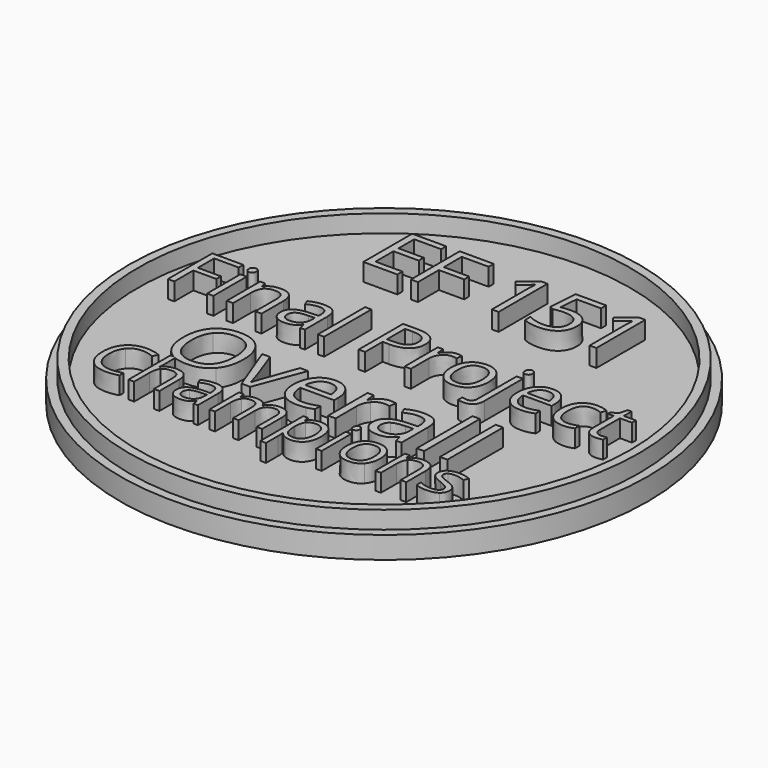
from build123d import *

# Parameters (mm, degrees)
F0_R           = 38.1
F1_DEPTH       = 3.175
F2_R           = 36.83
F2_R_2         = 35.56
F3_DEPTH       = 2.54
F4_TEXT_SIZE   = 12.3391885464
F4_TEXT_SIZE_2 = 11.2342395975
F4_W           = 1.0741905417
F4_H           = 10.0651032839
F4_W_2         = 0.8091592002
F4_H_2         = 5.3398270918
F5_DEPTH       = 2.54


# Not quite as in the source:
# - Text() gives the source's letters only with a copy of the font that has no kerning and outlines rounded to 1/6400 em; it was checked with that copy


with BuildPart() as f1:
    # F0 (on Top) → F1 (new body)
    with BuildSketch(Plane.XY):
        Circle(F0_R)
    extrude(amount=F1_DEPTH)

    # F2 (on face) → F3 (join)
    with BuildSketch(Plane.XY.offset(3.175)):
        Circle(F2_R)
        Circle(F2_R_2, mode=Mode.SUBTRACT)
    extrude(amount=F3_DEPTH)

    # F4 (on face) → F5 (join)
    with BuildSketch(Plane.XY.offset(3.175)):
        with Locations((-17.8262714532, 17.0286893845)):
            Text('EF 151', F4_TEXT_SIZE, font='Open Sans', text_align=(TextAlign.LEFT, TextAlign.BOTTOM))
        with Locations((-32.3159923422, 0)):
            Text('Final Project', F4_TEXT_SIZE_2, font='Open Sans', text_align=(TextAlign.LEFT, TextAlign.BOTTOM))
        with BuildLine():
            add(Edge.make_bspline(
                [(-12.2817855001, -10.0030932078), (-12.2817855001, -12.2735884376), (-13.4304863684, -13.5744145561)],
                knots=[0, 0, 0, 1, 1, 1], degree=2))
            add(Edge.make_bspline(
                [(-13.4263469058, -6.4328067252), (-12.2817855001, -7.7263887842), (-12.2817855001, -10.0030932078)],
                knots=[0, 0, 0, 1, 1, 1], degree=2))
            add(Edge.make_bspline(
                [(-16.6095936364, -5.1392246663), (-14.5709083115, -5.1392246663), (-13.4263469058, -6.4328067252)],
                knots=[0, 0, 0, 1, 1, 1], degree=2))
            add(Edge.make_bspline(
                [(-19.842513918, -6.410039681), (-18.7041617061, -5.1392246663), (-16.6095936364, -5.1392246663)],
                knots=[0, 0, 0, 1, 1, 1], degree=2))
            add(Edge.make_bspline(
                [(-20.9808661298, -9.9906748201), (-20.9808661298, -7.6808546957), (-19.842513918, -6.410039681)],
                knots=[0, 0, 0, 1, 1, 1], degree=2))
            add(Edge.make_bspline(
                [(-19.8456185149, -13.5971816003), (-20.9808661298, -12.3191225261), (-20.9808661298, -9.9906748201)],
                knots=[0, 0, 0, 1, 1, 1], degree=2))
            add(Edge.make_bspline(
                [(-18.9127607209, -14.3472838341), (-19.4400204931, -14.0538028919), (-19.8456185149, -13.5971816003)],
                knots=[0.6427228594, 0.6427228594, 0.6427228594, 1, 1, 1], degree=2))
            Line((-18.9127607209, -14.3472838341), (-18.5319283874, -14.3472838341))
            Line((-18.5319283874, -14.3472838341), (-18.5319283874, -14.5314262065))
            add(Edge.make_bspline(
                [(-16.6220120241, -14.8752406745), (-17.7051698515, -14.8752406745), (-18.5319283874, -14.5314262065)],
                knots=[0, 0, 0, 0.5186646031, 0.5186646031, 0.5186646031], degree=2))
            add(Edge.make_bspline(
                [(-13.4304863684, -13.5744145561), (-14.5791872367, -14.8752406745), (-16.6220120241, -14.8752406745)],
                knots=[0, 0, 0, 1, 1, 1], degree=2))
        make_face()
        with BuildLine():
            add(Edge.make_bspline(
                [(-19.8176771424, -10.0030932078), (-19.8176771424, -11.9238038489), (-18.9990984156, -12.9172748701)],
                knots=[0, 0, 0, 1, 1, 1], degree=2))
            add(Edge.make_bspline(
                [(-18.9990984156, -7.1158180523), (-19.8176771424, -8.1092890736), (-19.8176771424, -10.0030932078)],
                knots=[0, 0, 0, 1, 1, 1], degree=2))
            add(Edge.make_bspline(
                [(-16.6095936364, -6.1223470311), (-18.1805196887, -6.1223470311), (-18.9990984156, -7.1158180523)],
                knots=[0, 0, 0, 1, 1, 1], degree=2))
            add(Edge.make_bspline(
                [(-14.2459604983, -7.1085739928), (-15.0448767779, -6.1223470311), (-16.6095936364, -6.1223470311)],
                knots=[0, 0, 0, 1, 1, 1], degree=2))
            add(Edge.make_bspline(
                [(-13.4470442187, -10.0030932078), (-13.4470442187, -8.0948009545), (-14.2459604983, -7.1085739928)],
                knots=[0, 0, 0, 1, 1, 1], degree=2))
            add(Edge.make_bspline(
                [(-14.2490650953, -12.9214143327), (-13.4470442187, -11.9320827741), (-13.4470442187, -10.0030932078)],
                knots=[0, 0, 0, 1, 1, 1], degree=2))
            add(Edge.make_bspline(
                [(-16.6220120241, -13.9107458914), (-15.0510859718, -13.9107458914), (-14.2490650953, -12.9214143327)],
                knots=[0, 0, 0, 1, 1, 1], degree=2))
            add(Edge.make_bspline(
                [(-18.9990984156, -12.9172748701), (-18.1805196887, -13.9107458914), (-16.6220120241, -13.9107458914)],
                knots=[0, 0, 0, 1, 1, 1], degree=2))
        make_face(mode=Mode.SUBTRACT)
        with BuildLine():
            Line((-18.5319283874, -16.6422401784), (-18.5319283874, -14.5314262065))
            add(Edge.make_bspline(
                [(-18.5319283874, -14.5314262065), (-18.7296789602, -14.449189973), (-18.9127607209, -14.3472838341)],
                knots=[0.5186646031, 0.5186646031, 0.5186646031, 0.6427228594, 0.6427228594, 0.6427228594], degree=2))
            Line((-18.9127607209, -14.3472838341), (-19.3410875876, -14.3472838341))
            Line((-19.3410875876, -14.3472838341), (-19.3410875876, -21.9290587677))
            Line((-19.3410875876, -21.9290587677), (-18.5319283874, -21.9290587677))
            Line((-18.5319283874, -21.9290587677), (-18.5319283874, -19.1367579439))
            add(Edge.make_bspline(
                [(-18.144498597, -17.6369291374), (-18.5319283874, -18.0952967768), (-18.5319283874, -19.1367579439)],
                knots=[0, 0, 0, 1, 1, 1], degree=2))
            add(Edge.make_bspline(
                [(-16.9151690607, -17.1785614979), (-17.7570688065, -17.1785614979), (-18.144498597, -17.6369291374)],
                knots=[0, 0, 0, 1, 1, 1], degree=2))
            add(Edge.make_bspline(
                [(-15.9836225826, -17.5005101971), (-16.2806261041, -17.1785614979), (-16.9151690607, -17.1785614979)],
                knots=[0, 0, 0, 1, 1, 1], degree=2))
            add(Edge.make_bspline(
                [(-15.6866190611, -18.4741516624), (-15.6866190611, -17.8224588962), (-15.9836225826, -17.5005101971)],
                knots=[0, 0, 0, 1, 1, 1], degree=2))
            Line((-15.6866190611, -18.4741516624), (-15.6866190611, -21.9290587677))
            Line((-15.6866190611, -21.9290587677), (-14.877459861, -21.9290587677))
            Line((-14.877459861, -21.9290587677), (-14.877459861, -18.4460883376))
            add(Edge.make_bspline(
                [(-15.3677885092, -16.9673070247), (-14.877459861, -17.4326904953), (-14.877459861, -18.4460883376)],
                knots=[0, 0, 0, 1, 1, 1], degree=2))
            add(Edge.make_bspline(
                [(-16.8372153805, -16.501923554), (-15.8581171575, -16.501923554), (-15.3677885092, -16.9673070247)],
                knots=[0, 0, 0, 1, 1, 1], degree=2))
            add(Edge.make_bspline(
                [(-17.8428178547, -16.7233120057), (-17.4016000249, -16.501923554), (-16.8372153805, -16.501923554)],
                knots=[0, 0, 0, 1, 1, 1], degree=2))
            add(Edge.make_bspline(
                [(-18.5225739458, -17.3297916375), (-18.2840356845, -16.9447004574), (-17.8428178547, -16.7233120057)],
                knots=[0, 0, 0, 1, 1, 1], degree=2))
            Line((-18.5225739458, -17.3297916375), (-18.5709052275, -17.3297916375))
            add(Edge.make_bspline(
                [(-18.5319283874, -16.6422401784), (-18.5319283874, -17.0569537569), (-18.5709052275, -17.3297916375)],
                knots=[0, 0, 0, 1, 1, 1], degree=2))
        make_face()
        with BuildLine():
            add(Edge.make_bspline(
                [(-18.5319283874, -14.5314262065), (-18.7296789602, -14.449189973), (-18.9127607209, -14.3472838341)],
                knots=[0.5186646031, 0.5186646031, 0.5186646031, 0.6427228594, 0.6427228594, 0.6427228594], degree=2))
            Line((-18.5319283874, -14.5314262065), (-18.5319283874, -14.3472838341))
            Line((-18.5319283874, -14.3472838341), (-18.9127607209, -14.3472838341))
        make_face()
        with BuildLine():
            Line((-11.4745902953, -7.6560179201), (-8.7839396128, -14.744847603))
            Line((-8.7839396128, -14.744847603), (-7.5296824485, -14.744847603))
            Line((-7.5296824485, -14.744847603), (-4.839031766, -7.6560179201))
            Line((-4.839031766, -7.6560179201), (-5.9898023656, -7.6560179201))
            add(Edge.make_bspline(
                [(-7.6869820268, -12.3553428237), (-7.3082212, -11.2780476851), (-5.9898023656, -7.6560179201)],
                knots=[0, 0, 0, 1, 1, 1], degree=2))
            add(Edge.make_bspline(
                [(-8.1361137177, -13.774143626), (-8.0657428537, -13.4326379624), (-7.6869820268, -12.3553428237)],
                knots=[0, 0, 0, 1, 1, 1], degree=2))
            Line((-8.1361137177, -13.774143626), (-8.1878570001, -13.774143626))
            add(Edge.make_bspline(
                [(-8.7963580006, -11.8596421788), (-8.278925177, -13.3353605916), (-8.1878570001, -13.774143626)],
                knots=[0, 0, 0, 1, 1, 1], degree=2))
            Line((-8.7963580006, -11.8596421788), (-10.3238196957, -7.6560179201))
            Line((-10.3238196957, -7.6560179201), (-11.4745902953, -7.6560179201))
        make_face()
        with BuildLine():
            add(Edge.make_bspline(
                [(-0.7057783713, -14.8752406745), (-2.2767044237, -14.8752406745), (-3.1863513275, -13.9169550853)],
                knots=[0, 0, 0, 1, 1, 1], degree=2))
            add(Edge.make_bspline(
                [(0.5195025549, -14.7676146472), (0.0124183878, -14.8752406745), (-0.7057783713, -14.8752406745)],
                knots=[0, 0, 0, 1, 1, 1], degree=2))
            add(Edge.make_bspline(
                [(1.5957628279, -14.4157603272), (1.0265867219, -14.6599886199), (0.5195025549, -14.7676146472)],
                knots=[0, 0, 0, 1, 1, 1], degree=2))
            Line((1.5957628279, -14.4157603272), (1.5957628279, -13.4574747379))
            add(Edge.make_bspline(
                [(-0.6664534767, -13.9355826669), (0.478107929, -13.9355826669), (1.5957628279, -13.4574747379)],
                knots=[0, 0, 0, 1, 1, 1], degree=2))
            add(Edge.make_bspline(
                [(-2.3512147503, -13.2887916374), (-1.7530624062, -13.9355826669), (-0.6664534767, -13.9355826669)],
                knots=[0, 0, 0, 1, 1, 1], degree=2))
            add(Edge.make_bspline(
                [(-2.982482795, -11.3939526376), (-2.9493670943, -12.642000608), (-2.3512147503, -13.2887916374)],
                knots=[0, 0, 0, 1, 1, 1], degree=2))
            Line((-2.982482795, -11.3939526376), (1.9000133281, -11.3939526376))
            Line((1.9000133281, -11.3939526376), (1.9000133281, -10.715080773))
            add(Edge.make_bspline(
                [(1.1238640928, -8.4021560517), (1.9000133281, -9.2786872548), (1.9000133281, -10.715080773)],
                knots=[0, 0, 0, 1, 1, 1], degree=2))
            add(Edge.make_bspline(
                [(-0.9831223648, -7.5256248486), (0.3477148574, -7.5256248486), (1.1238640928, -8.4021560517)],
                knots=[0, 0, 0, 1, 1, 1], degree=2))
            add(Edge.make_bspline(
                [(-3.2515478633, -8.5346188546), (-2.4070974952, -7.5256248486), (-0.9831223648, -7.5256248486)],
                knots=[0, 0, 0, 1, 1, 1], degree=2))
            add(Edge.make_bspline(
                [(-4.0959982313, -11.2594201034), (-4.0959982313, -9.5436128605), (-3.2515478633, -8.5346188546)],
                knots=[0, 0, 0, 1, 1, 1], degree=2))
            add(Edge.make_bspline(
                [(-3.1863513275, -13.9169550853), (-4.0959982313, -12.958669496), (-4.0959982313, -11.2594201034)],
                knots=[0, 0, 0, 1, 1, 1], degree=2))
        make_face()
        with BuildLine():
            add(Edge.make_bspline(
                [(-0.9976104838, -8.4259579616), (-1.8503397771, -8.4259579616), (-2.3584588098, -8.9816808141)],
                knots=[0, 0, 0, 1, 1, 1], degree=2))
            add(Edge.make_bspline(
                [(0.2970064407, -8.9661578294), (-0.1552298471, -8.4259579616), (-0.9976104838, -8.4259579616)],
                knots=[0, 0, 0, 1, 1, 1], degree=2))
            add(Edge.make_bspline(
                [(0.7492427285, -10.5205260314), (0.7492427285, -9.5063576972), (0.2970064407, -8.9661578294)],
                knots=[0, 0, 0, 1, 1, 1], degree=2))
            Line((0.7492427285, -10.5205260314), (-2.9576460195, -10.5205260314))
            add(Edge.make_bspline(
                [(-2.3584588098, -8.9816808141), (-2.8665778425, -9.5374036666), (-2.9576460195, -10.5205260314)],
                knots=[0, 0, 0, 1, 1, 1], degree=2))
        make_face(mode=Mode.SUBTRACT)
        with BuildLine():
            add(Edge.make_bspline(
                [(6.9667155364, -7.5256248486), (7.4386142715, -7.5256248486), (7.8132356358, -7.6042746378)],
                knots=[0, 0, 0, 1, 1, 1], degree=2))
            add(Edge.make_bspline(
                [(5.7435043415, -7.9012810785), (6.3002620597, -7.5256248486), (6.9667155364, -7.5256248486)],
                knots=[0, 0, 0, 1, 1, 1], degree=2))
            add(Edge.make_bspline(
                [(4.7934976775, -8.9682275607), (5.1867466234, -8.2769373084), (5.7435043415, -7.9012810785)],
                knots=[0, 0, 0, 1, 1, 1], degree=2))
            Line((4.7934976775, -8.9682275607), (4.7417543951, -8.9682275607))
            Line((4.7417543951, -8.9682275607), (4.6175705175, -7.6560179201))
            Line((4.6175705175, -7.6560179201), (3.7317255235, -7.6560179201))
            Line((3.7317255235, -7.6560179201), (3.7317255235, -14.744847603))
            Line((3.7317255235, -14.744847603), (4.8059160652, -14.744847603))
            Line((4.8059160652, -14.744847603), (4.8059160652, -10.9406814841))
            add(Edge.make_bspline(
                [(5.4164867971, -9.2010723313), (4.8059160652, -9.8996066431), (4.8059160652, -10.9406814841)],
                knots=[0, 0, 0, 1, 1, 1], degree=2))
            add(Edge.make_bspline(
                [(6.8880657473, -8.5025380195), (6.0270575289, -8.5025380195), (5.4164867971, -9.2010723313)],
                knots=[0, 0, 0, 1, 1, 1], degree=2))
            add(Edge.make_bspline(
                [(7.6642149826, -8.5998153903), (7.2254319482, -8.5025380195), (6.8880657473, -8.5025380195)],
                knots=[0, 0, 0, 1, 1, 1], degree=2))
            Line((7.6642149826, -8.5998153903), (7.8132356358, -7.6042746378))
        make_face()
        with BuildLine():
            Line((13.2856051778, -13.7348187314), (13.4987875011, -14.744847603))
            Line((13.4987875011, -14.744847603), (14.2956340494, -14.744847603))
            Line((14.2956340494, -14.744847603), (14.2956340494, -9.905815837))
            add(Edge.make_bspline(
                [(13.6840284519, -8.1020450141), (14.2956340494, -8.6639770604), (14.2956340494, -9.905815837)],
                knots=[0, 0, 0, 1, 1, 1], degree=2))
            add(Edge.make_bspline(
                [(11.8057473024, -7.5401129677), (13.0724228545, -7.5401129677), (13.6840284519, -8.1020450141)],
                knots=[0, 0, 0, 1, 1, 1], degree=2))
            add(Edge.make_bspline(
                [(10.5525250037, -7.7015520086), (11.1765489889, -7.5401129677), (11.8057473024, -7.5401129677)],
                knots=[0, 0, 0, 1, 1, 1], degree=2))
            add(Edge.make_bspline(
                [(9.4048590011, -8.1465442369), (9.9285010185, -7.8629910496), (10.5525250037, -7.7015520086)],
                knots=[0, 0, 0, 1, 1, 1], degree=2))
            Line((9.4048590011, -8.1465442369), (9.7360160082, -8.9682275607))
            add(Edge.make_bspline(
                [(11.739515901, -8.4259579616), (10.853670907, -8.4259579616), (9.7360160082, -8.9682275607)],
                knots=[0, 0, 0, 1, 1, 1], degree=2))
            add(Edge.make_bspline(
                [(12.8882167693, -8.8233463701), (12.5301532554, -8.4259579616), (11.739515901, -8.4259579616)],
                knots=[0, 0, 0, 1, 1, 1], degree=2))
            add(Edge.make_bspline(
                [(13.2462802832, -10.0548364902), (13.2462802832, -9.2207347786), (12.8882167693, -8.8233463701)],
                knots=[0, 0, 0, 1, 1, 1], degree=2))
            Line((13.2462802832, -10.0548364902), (13.2462802832, -10.4956892559))
            Line((13.2462802832, -10.4956892559), (12.0437664012, -10.5350141505))
            add(Edge.make_bspline(
                [(8.6100821841, -12.7848120673), (8.6100821841, -10.6385007152), (12.0437664012, -10.5350141505)],
                knots=[0, 0, 0, 1, 1, 1], degree=2))
            add(Edge.make_bspline(
                [(9.2082345281, -14.3309013441), (8.6100821841, -13.7865620137), (8.6100821841, -12.7848120673)],
                knots=[0, 0, 0, 1, 1, 1], degree=2))
            add(Edge.make_bspline(
                [(10.8598801009, -14.8752406745), (9.8063868722, -14.8752406745), (9.2082345281, -14.3309013441)],
                knots=[0, 0, 0, 1, 1, 1], degree=2))
            add(Edge.make_bspline(
                [(12.1772640697, -14.6382564413), (11.6505174553, -14.8752406745), (10.8598801009, -14.8752406745)],
                knots=[0, 0, 0, 1, 1, 1], degree=2))
            add(Edge.make_bspline(
                [(13.2338618954, -13.7348187314), (12.7040106841, -14.4012722081), (12.1772640697, -14.6382564413)],
                knots=[0, 0, 0, 1, 1, 1], degree=2))
            Line((13.2338618954, -13.7348187314), (13.2856051778, -13.7348187314))
        make_face()
        with BuildLine():
            add(Edge.make_bspline(
                [(11.0730624242, -13.9873259493), (12.0768821019, -13.9873259493), (12.6491628048, -13.4378122906)],
                knots=[0, 0, 0, 1, 1, 1], degree=2))
            add(Edge.make_bspline(
                [(10.0878703282, -13.6841103147), (10.4397246482, -13.9873259493), (11.0730624242, -13.9873259493)],
                knots=[0, 0, 0, 1, 1, 1], degree=2))
            add(Edge.make_bspline(
                [(9.7360160082, -12.7972304551), (9.7360160082, -13.38089468), (10.0878703282, -13.6841103147)],
                knots=[0, 0, 0, 1, 1, 1], degree=2))
            add(Edge.make_bspline(
                [(10.3010526515, -11.7013077348), (9.7360160082, -12.0541969204), (9.7360160082, -12.7972304551)],
                knots=[0, 0, 0, 1, 1, 1], degree=2))
            add(Edge.make_bspline(
                [(12.147252966, -11.3028844606), (10.8660892948, -11.3484185491), (10.3010526515, -11.7013077348)],
                knots=[0, 0, 0, 1, 1, 1], degree=2))
            Line((12.147252966, -11.3028844606), (13.2214435077, -11.2594201034))
            Line((13.2214435077, -11.2594201034), (13.2214435077, -11.8989670734))
            add(Edge.make_bspline(
                [(12.6491628048, -13.4378122906), (13.2214435077, -12.888298632), (13.2214435077, -11.8989670734)],
                knots=[0, 0, 0, 1, 1, 1], degree=2))
        make_face(mode=Mode.SUBTRACT)
        with Locations((17.0432023425, -9.712295961)):
            Rectangle(F4_W, F4_H)
        with Locations((20.3940973079, -9.712295961)):
            Rectangle(F4_W, F4_H)
        with BuildLine():
            add(Edge.make_bspline(
                [(-22.465471089, -15.4448716509), (-23.6394535124, -15.4448716509), (-24.3192096035, -16.226747063)],
                knots=[0, 0, 0, 1, 1, 1], degree=2))
            add(Edge.make_bspline(
                [(-20.8471526886, -15.8237265365), (-21.6563118888, -15.4448716509), (-22.465471089, -15.4448716509)],
                knots=[0, 0, 0, 1, 1, 1], degree=2))
            Line((-20.8471526886, -15.8237265365), (-20.4963611278, -15.1127889734))
            add(Edge.make_bspline(
                [(-22.4545575737, -14.7043116893), (-21.3351427265, -14.7043116893), (-20.4963611278, -15.1127889734)],
                knots=[0, 0, 0, 1, 1, 1], degree=2))
            add(Edge.make_bspline(
                [(-24.2841304474, -15.1525453503), (-23.5069322561, -14.7043116893), (-22.4545575737, -14.7043116893)],
                knots=[0, 0, 0, 1, 1, 1], degree=2))
            add(Edge.make_bspline(
                [(-25.47292407, -16.4286470947), (-25.0613286387, -15.6007790113), (-24.2841304474, -15.1525453503)],
                knots=[0, 0, 0, 1, 1, 1], degree=2))
            add(Edge.make_bspline(
                [(-25.8845195013, -18.3572211422), (-25.8845195013, -17.2565151781), (-25.47292407, -16.4286470947)],
                knots=[0, 0, 0, 1, 1, 1], degree=2))
            add(Edge.make_bspline(
                [(-25.0293676298, -21.0715682858), (-25.8845195013, -20.1158561669), (-25.8845195013, -18.3572211422)],
                knots=[0, 0, 0, 1, 1, 1], degree=2))
            add(Edge.make_bspline(
                [(-22.6011104925, -22.0272804047), (-24.1742157583, -22.0272804047), (-25.0293676298, -21.0715682858)],
                knots=[0, 0, 0, 1, 1, 1], degree=2))
            add(Edge.make_bspline(
                [(-20.7738762292, -21.7482062297), (-21.5144361909, -22.0272804047), (-22.6011104925, -22.0272804047)],
                knots=[0, 0, 0, 1, 1, 1], degree=2))
            Line((-20.7738762292, -21.7482062297), (-20.7738762292, -21.0232370041))
            add(Edge.make_bspline(
                [(-22.4748255306, -21.2913976639), (-21.7295883481, -21.2913976639), (-20.7738762292, -21.0232370041)],
                knots=[0, 0, 0, 1, 1, 1], degree=2))
            add(Edge.make_bspline(
                [(-24.3433752443, -20.528231135), (-23.6877847941, -21.2913976639), (-22.4748255306, -21.2913976639)],
                knots=[0, 0, 0, 1, 1, 1], degree=2))
            add(Edge.make_bspline(
                [(-24.9989656946, -18.3681346574), (-24.9989656946, -19.7650646061), (-24.3433752443, -20.528231135)],
                knots=[0, 0, 0, 1, 1, 1], degree=2))
            add(Edge.make_bspline(
                [(-24.3192096035, -16.226747063), (-24.9989656946, -17.0086224752), (-24.9989656946, -18.3681346574)],
                knots=[0, 0, 0, 1, 1, 1], degree=2))
        make_face()
        with BuildLine():
            Line((-10.0942220456, -21.1682308492), (-9.9336374644, -21.9290587677))
            Line((-9.9336374644, -21.9290587677), (-9.3333941271, -21.9290587677))
            Line((-9.3333941271, -21.9290587677), (-9.3333941271, -18.2839446828))
            add(Edge.make_bspline(
                [(-9.7941003769, -16.9252120374), (-9.3333941271, -17.3485005207), (-9.3333941271, -18.2839446828)],
                knots=[0, 0, 0, 1, 1, 1], degree=2))
            add(Edge.make_bspline(
                [(-11.208959672, -16.501923554), (-10.2548066267, -16.501923554), (-9.7941003769, -16.9252120374)],
                knots=[0, 0, 0, 1, 1, 1], degree=2))
            add(Edge.make_bspline(
                [(-12.1529787389, -16.6235312951), (-11.6829180475, -16.501923554), (-11.208959672, -16.501923554)],
                knots=[0, 0, 0, 1, 1, 1], degree=2))
            add(Edge.make_bspline(
                [(-13.017485052, -16.9587321199), (-12.6230394304, -16.7451390362), (-12.1529787389, -16.6235312951)],
                knots=[0, 0, 0, 1, 1, 1], degree=2))
            Line((-13.017485052, -16.9587321199), (-12.7680332755, -17.5776843404))
            add(Edge.make_bspline(
                [(-11.2588500273, -17.1692070563), (-11.9261335296, -17.1692070563), (-12.7680332755, -17.5776843404)],
                knots=[0, 0, 0, 1, 1, 1], degree=2))
            add(Edge.make_bspline(
                [(-10.3935641774, -17.4685491882), (-10.6632839108, -17.1692070563), (-11.2588500273, -17.1692070563)],
                knots=[0, 0, 0, 1, 1, 1], degree=2))
            add(Edge.make_bspline(
                [(-10.123844444, -18.3961979822), (-10.123844444, -17.7678913201), (-10.3935641774, -17.4685491882)],
                knots=[0, 0, 0, 1, 1, 1], degree=2))
            Line((-10.123844444, -18.3961979822), (-10.123844444, -18.7282806598))
            Line((-10.123844444, -18.7282806598), (-11.0296662076, -18.7579030582))
            add(Edge.make_bspline(
                [(-13.6161693158, -20.4526160652), (-13.6161693158, -18.8358567384), (-11.0296662076, -18.7579030582)],
                knots=[0, 0, 0, 1, 1, 1], degree=2))
            add(Edge.make_bspline(
                [(-13.1655970444, -21.617244047), (-13.6161693158, -21.2072076893), (-13.6161693158, -20.4526160652)],
                knots=[0, 0, 0, 1, 1, 1], degree=2))
            add(Edge.make_bspline(
                [(-11.9214563088, -22.0272804047), (-12.715024773, -22.0272804047), (-13.1655970444, -21.617244047)],
                knots=[0, 0, 0, 1, 1, 1], degree=2))
            add(Edge.make_bspline(
                [(-10.9291059602, -21.8487664771), (-11.3258901923, -22.0272804047), (-11.9214563088, -22.0272804047)],
                knots=[0, 0, 0, 1, 1, 1], degree=2))
            add(Edge.make_bspline(
                [(-10.1331988856, -21.1682308492), (-10.5323217281, -21.6702525495), (-10.9291059602, -21.8487664771)],
                knots=[0, 0, 0, 1, 1, 1], degree=2))
            Line((-10.1331988856, -21.1682308492), (-10.0942220456, -21.1682308492))
        make_face()
        with BuildLine():
            add(Edge.make_bspline(
                [(-11.7608717277, -21.3584378288), (-11.00472103, -21.3584378288), (-10.5736371786, -20.9445037871)],
                knots=[0, 0, 0, 1, 1, 1], degree=2))
            add(Edge.make_bspline(
                [(-12.5029907629, -21.1300335459), (-12.2379482503, -21.3584378288), (-11.7608717277, -21.3584378288)],
                knots=[0, 0, 0, 1, 1, 1], degree=2))
            add(Edge.make_bspline(
                [(-12.7680332755, -20.4619705068), (-12.7680332755, -20.901629263), (-12.5029907629, -21.1300335459)],
                knots=[0, 0, 0, 1, 1, 1], degree=2))
            add(Edge.make_bspline(
                [(-12.3424061817, -19.6364410338), (-12.7680332755, -19.9022630832), (-12.7680332755, -20.4619705068)],
                knots=[0, 0, 0, 1, 1, 1], degree=2))
            add(Edge.make_bspline(
                [(-10.9517125275, -19.3363193651), (-11.916779088, -19.3706189844), (-12.3424061817, -19.6364410338)],
                knots=[0, 0, 0, 1, 1, 1], degree=2))
            Line((-10.9517125275, -19.3363193651), (-10.1425533273, -19.3035788195))
            Line((-10.1425533273, -19.3035788195), (-10.1425533273, -19.7853325629))
            add(Edge.make_bspline(
                [(-10.5736371786, -20.9445037871), (-10.1425533273, -20.5305697454), (-10.1425533273, -19.7853325629)],
                knots=[0, 0, 0, 1, 1, 1], degree=2))
        make_face(mode=Mode.SUBTRACT)
        with BuildLine():
            Line((-0.8613881659, -18.4554427792), (-0.8613881659, -21.9290587677))
            Line((-0.8613881659, -21.9290587677), (-0.0537880393, -21.9290587677))
            Line((-0.0537880393, -21.9290587677), (-0.0537880393, -18.4460883376))
            add(Edge.make_bspline(
                [(-0.5043603107, -16.9563935095), (-0.0537880393, -17.4217769801), (-0.0537880393, -18.4460883376)],
                knots=[0, 0, 0, 1, 1, 1], degree=2))
            add(Edge.make_bspline(
                [(-1.8607543457, -16.4910100388), (-0.9549325821, -16.4910100388), (-0.5043603107, -16.9563935095)],
                knots=[0, 0, 0, 1, 1, 1], degree=2))
            add(Edge.make_bspline(
                [(-2.893640608, -16.7350050578), (-2.4407297262, -16.4910100388), (-1.8607543457, -16.4910100388)],
                knots=[0, 0, 0, 1, 1, 1], degree=2))
            add(Edge.make_bspline(
                [(-3.5850897511, -17.398390876), (-3.3465514898, -16.9790000767), (-2.893640608, -16.7350050578)],
                knots=[0, 0, 0, 1, 1, 1], degree=2))
            Line((-3.5850897511, -17.398390876), (-3.6240665912, -17.398390876))
            add(Edge.make_bspline(
                [(-5.2610938749, -16.4910100388), (-4.0091577713, -16.4910100388), (-3.6240665912, -17.398390876)],
                knots=[0, 0, 0, 1, 1, 1], degree=2))
            add(Edge.make_bspline(
                [(-6.1941994265, -16.7108394169), (-5.7771472376, -16.4910100388), (-5.2610938749, -16.4910100388)],
                knots=[0, 0, 0, 1, 1, 1], degree=2))
            add(Edge.make_bspline(
                [(-6.8404354352, -17.3204371959), (-6.6112516154, -16.930668795), (-6.1941994265, -16.7108394169)],
                knots=[0, 0, 0, 1, 1, 1], degree=2))
            Line((-6.8404354352, -17.3204371959), (-6.8794122752, -17.3204371959))
            Line((-6.8794122752, -17.3204371959), (-7.0103744579, -16.5892316758))
            Line((-7.0103744579, -16.5892316758), (-7.6683035186, -16.5892316758))
            Line((-7.6683035186, -16.5892316758), (-7.6683035186, -21.9290587677))
            Line((-7.6683035186, -21.9290587677), (-6.8591443184, -21.9290587677))
            Line((-6.8591443184, -21.9290587677), (-6.8591443184, -19.1274035023))
            add(Edge.make_bspline(
                [(-6.5060141472, -17.6338109902), (-6.8591443184, -18.0890604824), (-6.8591443184, -19.1274035023)],
                knots=[0, 0, 0, 1, 1, 1], degree=2))
            add(Edge.make_bspline(
                [(-5.3936151311, -17.1785614979), (-6.152883976, -17.1785614979), (-6.5060141472, -17.6338109902)],
                knots=[0, 0, 0, 1, 1, 1], degree=2))
            add(Edge.make_bspline(
                [(-4.5408018701, -17.4973920499), (-4.8136397507, -17.1785614979), (-5.3936151311, -17.1785614979)],
                knots=[0, 0, 0, 1, 1, 1], degree=2))
            add(Edge.make_bspline(
                [(-4.2679639895, -18.4554427792), (-4.2679639895, -17.8162226018), (-4.5408018701, -17.4973920499)],
                knots=[0, 0, 0, 1, 1, 1], degree=2))
            Line((-4.2679639895, -18.4554427792), (-4.2679639895, -21.9290587677))
            Line((-4.2679639895, -21.9290587677), (-3.4588047893, -21.9290587677))
            Line((-3.4588047893, -21.9290587677), (-3.4588047893, -18.9465509643))
            add(Edge.make_bspline(
                [(-3.0978792501, -17.6119839597), (-3.4588047893, -18.0454064215), (-3.4588047893, -18.9465509643)],
                knots=[0, 0, 0, 1, 1, 1], degree=2))
            add(Edge.make_bspline(
                [(-1.9823620868, -17.1785614979), (-2.7369537109, -17.1785614979), (-3.0978792501, -17.6119839597)],
                knots=[0, 0, 0, 1, 1, 1], degree=2))
            add(Edge.make_bspline(
                [(-1.1342260465, -17.4973920499), (-1.4070639271, -17.1785614979), (-1.9823620868, -17.1785614979)],
                knots=[0, 0, 0, 1, 1, 1], degree=2))
            add(Edge.make_bspline(
                [(-0.8613881659, -18.4554427792), (-0.8613881659, -17.8162226018), (-1.1342260465, -17.4973920499)],
                knots=[0, 0, 0, 1, 1, 1], degree=2))
        make_face()
        with BuildLine():
            add(Edge.make_bspline(
                [(4.0980249667, -22.0272804047), (3.5757353095, -22.0272804047), (3.1446514582, -21.8347348147)],
                knots=[0, 0, 0, 1, 1, 1], degree=2))
            add(Edge.make_bspline(
                [(5.7280364191, -21.2984134951), (5.1410452074, -22.0272804047), (4.0980249667, -22.0272804047)],
                knots=[0, 0, 0, 1, 1, 1], degree=2))
            add(Edge.make_bspline(
                [(6.3150276308, -19.2536884641), (6.3150276308, -20.5695465855), (5.7280364191, -21.2984134951)],
                knots=[0, 0, 0, 1, 1, 1], degree=2))
            add(Edge.make_bspline(
                [(5.7373908607, -17.217538338), (6.3150276308, -17.9440666372), (6.3150276308, -19.2536884641)],
                knots=[0, 0, 0, 1, 1, 1], degree=2))
            add(Edge.make_bspline(
                [(4.0980249667, -16.4910100388), (5.1597540906, -16.4910100388), (5.7373908607, -17.217538338)],
                knots=[0, 0, 0, 1, 1, 1], degree=2))
            add(Edge.make_bspline(
                [(3.1477696054, -16.6858942393), (3.5617036471, -16.4910100388), (4.0980249667, -16.4910100388)],
                knots=[0, 0, 0, 1, 1, 1], degree=2))
            add(Edge.make_bspline(
                [(2.422020843, -17.3204371959), (2.7338355637, -16.8807784397), (3.1477696054, -16.6858942393)],
                knots=[0, 0, 0, 1, 1, 1], degree=2))
            Line((2.422020843, -17.3204371959), (2.3830440029, -17.3204371959))
            Line((2.3830440029, -17.3204371959), (2.2707907034, -16.5892316758))
            Line((2.2707907034, -16.5892316758), (1.6128616428, -16.5892316758))
            Line((1.6128616428, -16.5892316758), (1.6128616428, -24.3269139698))
            Line((1.6128616428, -24.3269139698), (2.422020843, -24.3269139698))
            Line((2.422020843, -24.3269139698), (2.422020843, -22.1286201889))
            add(Edge.make_bspline(
                [(2.362776046, -21.2415073085), (2.422020843, -21.7092293896), (2.422020843, -22.1286201889)],
                knots=[0, 0, 0, 1, 1, 1], degree=2))
            Line((2.362776046, -21.2415073085), (2.422020843, -21.2415073085))
            add(Edge.make_bspline(
                [(3.1446514582, -21.8347348147), (2.7135676068, -21.6421892246), (2.422020843, -21.2415073085)],
                knots=[0, 0, 0, 1, 1, 1], degree=2))
        make_face()
        with BuildLine():
            add(Edge.make_bspline(
                [(3.9810944464, -17.1785614979), (3.1625808046, -17.1785614979), (2.7969780446, -17.6314723797)],
                knots=[0, 0, 0, 1, 1, 1], degree=2))
            add(Edge.make_bspline(
                [(5.0841390209, -17.7117646703), (4.6920320096, -17.1785614979), (3.9810944464, -17.1785614979)],
                knots=[0, 0, 0, 1, 1, 1], degree=2))
            add(Edge.make_bspline(
                [(5.4762460321, -19.2443340225), (5.4762460321, -18.2449678427), (5.0841390209, -17.7117646703)],
                knots=[0, 0, 0, 1, 1, 1], degree=2))
            add(Edge.make_bspline(
                [(5.0841390209, -20.7885964267), (5.4762460321, -20.2281094663), (5.4762460321, -19.2443340225)],
                knots=[0, 0, 0, 1, 1, 1], degree=2))
            add(Edge.make_bspline(
                [(3.9998033297, -21.3490833872), (4.6920320096, -21.3490833872), (5.0841390209, -20.7885964267)],
                knots=[0, 0, 0, 1, 1, 1], degree=2))
            add(Edge.make_bspline(
                [(2.7969780446, -20.8642114965), (3.1719352462, -21.3490833872), (3.9998033297, -21.3490833872)],
                knots=[0, 0, 0, 1, 1, 1], degree=2))
            add(Edge.make_bspline(
                [(2.422020843, -19.2536884641), (2.422020843, -20.3793396058), (2.7969780446, -20.8642114965)],
                knots=[0, 0, 0, 1, 1, 1], degree=2))
            Line((2.422020843, -19.2536884641), (2.422020843, -19.0743949997))
            add(Edge.make_bspline(
                [(2.7969780446, -17.6314723797), (2.4313752846, -18.0843832616), (2.422020843, -19.0743949997)],
                knots=[0, 0, 0, 1, 1, 1], degree=2))
        make_face(mode=Mode.SUBTRACT)
        with Locations((8.1321279156, -19.2591452218)):
            Rectangle(F4_W_2, F4_H_2)
        with BuildLine():
            add(Edge.make_bspline(
                [(7.658949077, -15.1424113718), (7.658949077, -14.8648962704), (7.7953680173, -14.7354931613)],
                knots=[0, 0, 0, 1, 1, 1], degree=2))
            add(Edge.make_bspline(
                [(7.7953680173, -15.5493295823), (7.658949077, -15.4152492524), (7.658949077, -15.1424113718)],
                knots=[0, 0, 0, 1, 1, 1], degree=2))
            add(Edge.make_bspline(
                [(8.1375846732, -15.6834099122), (7.9317869576, -15.6834099122), (7.7953680173, -15.5493295823)],
                knots=[0, 0, 0, 1, 1, 1], degree=2))
            add(Edge.make_bspline(
                [(8.4735650348, -15.5493295823), (8.3324688737, -15.6834099122), (8.1375846732, -15.6834099122)],
                knots=[0, 0, 0, 1, 1, 1], degree=2))
            add(Edge.make_bspline(
                [(8.6146611959, -15.1424113718), (8.6146611959, -15.4152492524), (8.4735650348, -15.5493295823)],
                knots=[0, 0, 0, 1, 1, 1], degree=2))
            add(Edge.make_bspline(
                [(8.4735650348, -14.7378317717), (8.6146611959, -14.8695734912), (8.6146611959, -15.1424113718)],
                knots=[0, 0, 0, 1, 1, 1], degree=2))
            add(Edge.make_bspline(
                [(8.1375846732, -14.6060900522), (8.3324688737, -14.6060900522), (8.4735650348, -14.7378317717)],
                knots=[0, 0, 0, 1, 1, 1], degree=2))
            add(Edge.make_bspline(
                [(7.7953680173, -14.7354931613), (7.9317869576, -14.6060900522), (8.1375846732, -14.6060900522)],
                knots=[0, 0, 0, 1, 1, 1], degree=2))
        make_face()
        with BuildLine():
            add(Edge.make_bspline(
                [(14.8603100513, -19.2536884641), (14.8603100513, -20.5601921438), (14.2031605275, -21.2937362743)],
                knots=[0, 0, 0, 1, 1, 1], degree=2))
            add(Edge.make_bspline(
                [(14.2000423803, -17.2370267581), (14.8603100513, -17.9830434773), (14.8603100513, -19.2536884641)],
                knots=[0, 0, 0, 1, 1, 1], degree=2))
            add(Edge.make_bspline(
                [(12.4203598619, -16.4910100388), (13.5397747092, -16.4910100388), (14.2000423803, -17.2370267581)],
                knots=[0, 0, 0, 1, 1, 1], degree=2))
            add(Edge.make_bspline(
                [(10.6071572611, -17.2198769484), (11.2604091009, -16.4910100388), (12.4203598619, -16.4910100388)],
                knots=[0, 0, 0, 1, 1, 1], degree=2))
            add(Edge.make_bspline(
                [(9.9539054212, -19.2536884641), (9.9539054212, -17.9487438581), (10.6071572611, -17.2198769484)],
                knots=[0, 0, 0, 1, 1, 1], degree=2))
            add(Edge.make_bspline(
                [(10.2563657003, -20.7254539458), (9.9539054212, -20.0971472836), (9.9539054212, -19.2536884641)],
                knots=[0, 0, 0, 1, 1, 1], degree=2))
            add(Edge.make_bspline(
                [(11.1138561822, -21.6905205063), (10.5588259794, -21.353760608), (10.2563657003, -20.7254539458)],
                knots=[0, 0, 0, 1, 1, 1], degree=2))
            add(Edge.make_bspline(
                [(12.3860602426, -22.0272804047), (11.668886385, -22.0272804047), (11.1138561822, -21.6905205063)],
                knots=[0, 0, 0, 1, 1, 1], degree=2))
            add(Edge.make_bspline(
                [(14.2031605275, -21.2937362743), (13.5460110036, -22.0272804047), (12.3860602426, -22.0272804047)],
                knots=[0, 0, 0, 1, 1, 1], degree=2))
        make_face()
        with BuildLine():
            add(Edge.make_bspline(
                [(10.7926870199, -19.2536884641), (10.7926870199, -20.2779998216), (11.2019438408, -20.8135416044)],
                knots=[0, 0, 0, 1, 1, 1], degree=2))
            add(Edge.make_bspline(
                [(11.19726662, -17.7000716183), (10.7926870199, -18.2215817387), (10.7926870199, -19.2536884641)],
                knots=[0, 0, 0, 1, 1, 1], degree=2))
            add(Edge.make_bspline(
                [(12.3954146843, -17.1785614979), (11.6018462201, -17.1785614979), (11.19726662, -17.7000716183)],
                knots=[0, 0, 0, 1, 1, 1], degree=2))
            add(Edge.make_bspline(
                [(13.6114920949, -17.7070874495), (13.1998966636, -17.1785614979), (12.3954146843, -17.1785614979)],
                knots=[0, 0, 0, 1, 1, 1], degree=2))
            add(Edge.make_bspline(
                [(14.0230875263, -19.2536884641), (14.0230875263, -18.2356134011), (13.6114920949, -17.7070874495)],
                knots=[0, 0, 0, 1, 1, 1], degree=2))
            add(Edge.make_bspline(
                [(13.6114920949, -20.8158802148), (14.0230875263, -20.2826770424), (14.0230875263, -19.2536884641)],
                knots=[0, 0, 0, 1, 1, 1], degree=2))
            add(Edge.make_bspline(
                [(12.4047691259, -21.3490833872), (13.1998966636, -21.3490833872), (13.6114920949, -20.8158802148)],
                knots=[0, 0, 0, 1, 1, 1], degree=2))
            add(Edge.make_bspline(
                [(11.2019438408, -20.8135416044), (11.6112006617, -21.3490833872), (12.4047691259, -21.3490833872)],
                knots=[0, 0, 0, 1, 1, 1], degree=2))
        make_face(mode=Mode.SUBTRACT)
        with BuildLine():
            Line((19.933535557, -18.4741516624), (19.933535557, -21.9290587677))
            Line((19.933535557, -21.9290587677), (20.7426947571, -21.9290587677))
            Line((20.7426947571, -21.9290587677), (20.7426947571, -18.4460883376))
            add(Edge.make_bspline(
                [(20.2554842561, -16.9563935095), (20.7426947571, -17.4217769801), (20.7426947571, -18.4460883376)],
                knots=[0, 0, 0, 1, 1, 1], degree=2))
            add(Edge.make_bspline(
                [(18.8032071944, -16.4910100388), (19.768273755, -16.4910100388), (20.2554842561, -16.9563935095)],
                knots=[0, 0, 0, 1, 1, 1], degree=2))
            add(Edge.make_bspline(
                [(17.8046205514, -16.7085008065), (18.2528542124, -16.4910100388), (18.8032071944, -16.4910100388)],
                knots=[0, 0, 0, 1, 1, 1], degree=2))
            add(Edge.make_bspline(
                [(17.1069351139, -17.3204371959), (17.3563868904, -16.9259915742), (17.8046205514, -16.7085008065)],
                knots=[0, 0, 0, 1, 1, 1], degree=2))
            Line((17.1069351139, -17.3204371959), (17.0679582738, -17.3204371959))
            Line((17.0679582738, -17.3204371959), (16.9369960911, -16.5892316758))
            Line((16.9369960911, -16.5892316758), (16.2790670305, -16.5892316758))
            Line((16.2790670305, -16.5892316758), (16.2790670305, -21.9290587677))
            Line((16.2790670305, -21.9290587677), (17.0882262307, -21.9290587677))
            Line((17.0882262307, -21.9290587677), (17.0882262307, -19.1274035023))
            add(Edge.make_bspline(
                [(17.4779946315, -17.6314723797), (17.0882262307, -18.0843832616), (17.0882262307, -19.1274035023)],
                knots=[0, 0, 0, 1, 1, 1], degree=2))
            add(Edge.make_bspline(
                [(18.7049855574, -17.1785614979), (17.8677630324, -17.1785614979), (17.4779946315, -17.6314723797)],
                knots=[0, 0, 0, 1, 1, 1], degree=2))
            add(Edge.make_bspline(
                [(19.6365320355, -17.5005101971), (19.339528514, -17.1785614979), (18.7049855574, -17.1785614979)],
                knots=[0, 0, 0, 1, 1, 1], degree=2))
            add(Edge.make_bspline(
                [(19.933535557, -18.4741516624), (19.933535557, -17.8224588962), (19.6365320355, -17.5005101971)],
                knots=[0, 0, 0, 1, 1, 1], degree=2))
        make_face()
        with BuildLine():
            add(Edge.make_bspline(
                [(25.8471017349, -20.472884022), (25.8471017349, -21.2181212045), (25.292071532, -21.6227008046)],
                knots=[0, 0, 0, 1, 1, 1], degree=2))
            add(Edge.make_bspline(
                [(25.5134599837, -19.5904483625), (25.8471017349, -19.9412399233), (25.8471017349, -20.472884022)],
                knots=[0, 0, 0, 1, 1, 1], degree=2))
            add(Edge.make_bspline(
                [(24.2303424081, -18.8935424617), (25.1798182326, -19.2396568017), (25.5134599837, -19.5904483625)],
                knots=[0, 0, 0, 1, 1, 1], degree=2))
            add(Edge.make_bspline(
                [(23.294898246, -18.4983173033), (23.5381137281, -18.6347362436), (24.2303424081, -18.8935424617)],
                knots=[0, 0, 0, 1, 1, 1], degree=2))
            add(Edge.make_bspline(
                [(22.9417680748, -18.2114477602), (23.0516827639, -18.361898363), (23.294898246, -18.4983173033)],
                knots=[0, 0, 0, 1, 1, 1], degree=2))
            add(Edge.make_bspline(
                [(22.8318533858, -17.8458450002), (22.8318533858, -18.0609971575), (22.9417680748, -18.2114477602)],
                knots=[0, 0, 0, 1, 1, 1], degree=2))
            add(Edge.make_bspline(
                [(23.1241796864, -17.3492800575), (22.8318533858, -17.5293530587), (22.8318533858, -17.8458450002)],
                knots=[0, 0, 0, 1, 1, 1], degree=2))
            add(Edge.make_bspline(
                [(23.9918041467, -17.1692070563), (23.4165059871, -17.1692070563), (23.1241796864, -17.3492800575)],
                knots=[0, 0, 0, 1, 1, 1], degree=2))
            add(Edge.make_bspline(
                [(25.4479788924, -17.4997306603), (24.6450559866, -17.1692070563), (23.9918041467, -17.1692070563)],
                knots=[0, 0, 0, 1, 1, 1], degree=2))
            Line((25.4479788924, -17.4997306603), (25.736407509, -16.8418015996))
            add(Edge.make_bspline(
                [(24.0494898701, -16.4910100388), (24.9116575728, -16.4910100388), (25.736407509, -16.8418015996)],
                knots=[0, 0, 0, 1, 1, 1], degree=2))
            add(Edge.make_bspline(
                [(22.5933151244, -16.8690853877), (23.1249592232, -16.4910100388), (24.0494898701, -16.4910100388)],
                knots=[0, 0, 0, 1, 1, 1], degree=2))
            add(Edge.make_bspline(
                [(22.0616710257, -17.9004125763), (22.0616710257, -17.2471607365), (22.5933151244, -16.8690853877)],
                knots=[0, 0, 0, 1, 1, 1], degree=2))
            add(Edge.make_bspline(
                [(22.2152397756, -18.5279397017), (22.0616710257, -18.2652357996), (22.0616710257, -17.9004125763)],
                knots=[0, 0, 0, 1, 1, 1], degree=2))
            add(Edge.make_bspline(
                [(22.6829618566, -18.9980003932), (22.3688085255, -18.7906436039), (22.2152397756, -18.5279397017)],
                knots=[0, 0, 0, 1, 1, 1], degree=2))
            add(Edge.make_bspline(
                [(23.7423523702, -19.4828722838), (22.9971151877, -19.2053571824), (22.6829618566, -18.9980003932)],
                knots=[0, 0, 0, 1, 1, 1], degree=2))
            add(Edge.make_bspline(
                [(24.7978451997, -20.0067210146), (24.5281254663, -19.7853325629), (23.7423523702, -19.4828722838)],
                knots=[0, 0, 0, 1, 1, 1], degree=2))
            add(Edge.make_bspline(
                [(25.0675649331, -20.539924187), (25.0675649331, -20.2281094663), (24.7978451997, -20.0067210146)],
                knots=[0, 0, 0, 1, 1, 1], degree=2))
            add(Edge.make_bspline(
                [(24.7269073508, -21.1565377972), (25.0675649331, -20.9546377655), (25.0675649331, -20.539924187)],
                knots=[0, 0, 0, 1, 1, 1], degree=2))
            add(Edge.make_bspline(
                [(23.7532658854, -21.3584378288), (24.3862497684, -21.3584378288), (24.7269073508, -21.1565377972)],
                knots=[0, 0, 0, 1, 1, 1], degree=2))
            add(Edge.make_bspline(
                [(22.9027912347, -21.2469640662), (23.3432295277, -21.3584378288), (23.7532658854, -21.3584378288)],
                knots=[0, 0, 0, 1, 1, 1], degree=2))
            add(Edge.make_bspline(
                [(22.0772617617, -20.9406061031), (22.4623529418, -21.1354903035), (22.9027912347, -21.2469640662)],
                knots=[0, 0, 0, 1, 1, 1], degree=2))
            Line((22.0772617617, -20.9406061031), (22.0772617617, -21.6905205063))
            add(Edge.make_bspline(
                [(23.7329979286, -22.0272804047), (22.6712688046, -22.0272804047), (22.0772617617, -21.6905205063)],
                knots=[0, 0, 0, 1, 1, 1], degree=2))
            add(Edge.make_bspline(
                [(25.292071532, -21.6227008046), (24.7370413292, -22.0272804047), (23.7329979286, -22.0272804047)],
                knots=[0, 0, 0, 1, 1, 1], degree=2))
        make_face()
    extrude(amount=F5_DEPTH)


solid = f1.part
